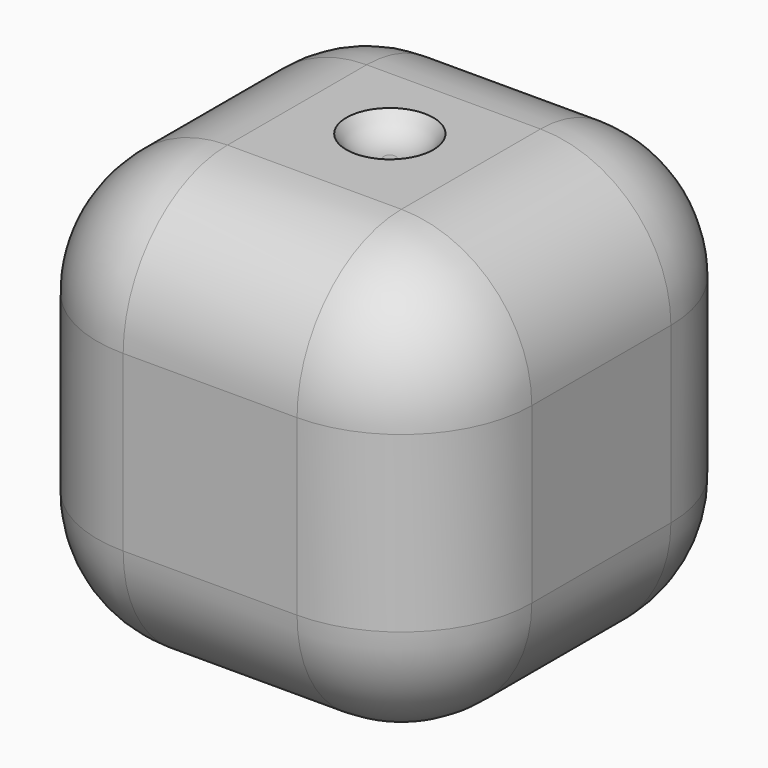
from build123d import *

# Parameters (mm, degrees)
F0_W     = 50.8
F0_H     = 50.8
F1_DEPTH = 50.8
F2_R     = 15.24
F3_R     = 5.08
F4_DEPTH = 2.54


# Not quite as in the source:
# - a fillet or chamfer that OpenCascade refuses, or shapes differently, is made with other operations: its cross-section is extruded or revolved along the edge and cut away or added


with BuildPart() as f1:
    # F0 (on Top) → F1 (new body)
    with BuildSketch(Plane.XY):
        with Locations((25.4, 25.4)):
            Rectangle(F0_W, F0_H)
    extrude(amount=F1_DEPTH)

    # F2
    f2_edges = [f1.edges().sort_by_distance(p)[0] for p in [
        (50.8, 25.4, 50.8),
        (25.4, 0, 50.8),
        (50.8, 0, 25.4),
        (50.8, 50.8, 25.4),
        (50.8, 25.4, 0),
        (25.4, 0, 0),
        (0, 0, 25.4),
        (0, 25.4, 50.8),
        (25.4, 50.8, 50.8),
        (25.4, 50.8, 0),
        (0, 25.4, 0),
        (0, 50.8, 25.4),
    ]]
    fillet(f2_edges, radius=F2_R)

    # F3 (on face) → F4 (cut)
    with BuildSketch(Plane.XY.offset(50.8)):
        with Locations((25.4, 26.2519493699)):
            Circle(F3_R)
    extrude(amount=-F4_DEPTH, mode=Mode.SUBTRACT)

    # F5: fillet of radius 5.08 on 1 edges, made by hand

    # F5_s1 → F5_t2 (revolve)
    with BuildSketch(Plane.XZ.offset(-26.2519493699)):
        with BuildLine():
            ThreePointArc((30.48, 50.8), (28.6205909488, 48.9405909488), (26.0805909488, 48.26))
            Line((26.0805909488, 48.26), (30.48, 48.26))
            Line((30.48, 48.26), (30.48, 50.8))
        make_face()
    revolve(axis=Axis((25.4, 26.2519493699, 48.26), (0, 0, 1)))


solid = f1.part
